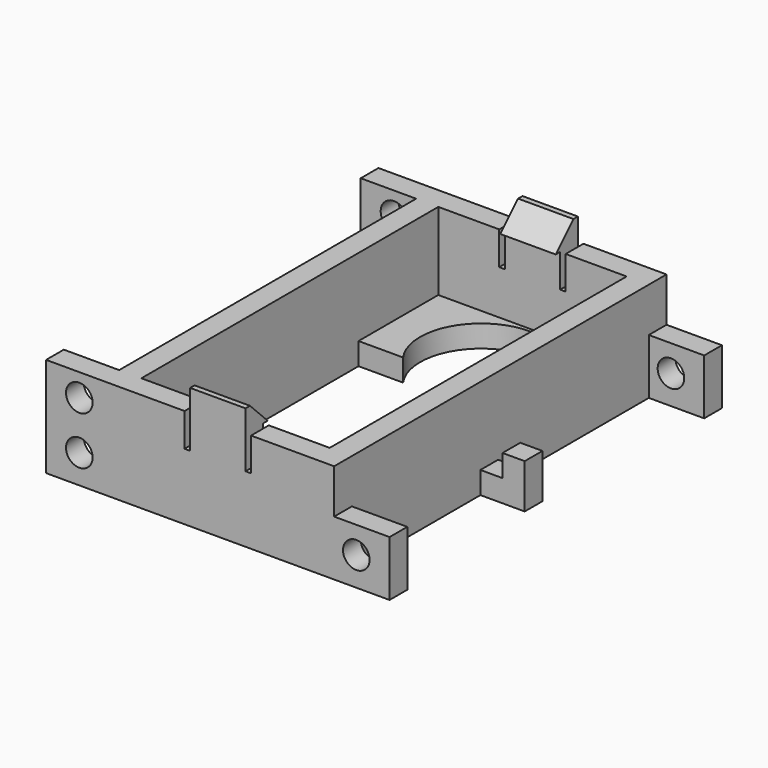
from build123d import *

# Parameters (mm, degrees)
F1_DEPTH  = 2
F2_DEPTH  = 9
F3_W      = 2
F3_H      = 5
F3_H_2    = 4
F4_DEPTH  = 5
F5_W      = 2
F5_H      = 5
F6_DEPTH  = 5
F7_R      = 1.2
F8_DEPTH  = 40
F11_DEPTH = 1
F12_W     = 5
F12_H     = 2
F12_H_2   = 0.5
F13_DEPTH = 2
F14_SIZE  = 1.99999
F12_W_2   = 0.5
F15_DEPTH = 3


# Not quite as in the source:
# - a fillet or chamfer is up to 0.001 mm smaller than in the source, because OpenCascade refuses the exact size


with BuildPart() as f1:
    # F0 (on Top) → F1 (new body)
    with BuildSketch(Plane.XY):
        Polygon((-5.1606558692, 9.7513413054), (-11.6606558692, 9.7513413054), (-11.6606558692, -27.7486586946), (-5.1606558692, -27.7486586946), (2.8393441308, -27.7486586946), (9.3393441308, -27.7486586946), (9.3393441308, 9.7513413054), (2.8393441308, 9.7513413054), align=None)
        Polygon((-9.6606558692, -1.2486586946), (-9.6606558692, 7.7513413054), (7.3393441308, 7.7513413054), (7.3393441308, -1.2486586946), (7.3393441308, -16.7486586946), (7.3393441308, -25.7486586946), (-9.6606558692, -25.7486586946), (-9.6606558692, -16.7486586946), align=None, mode=Mode.SUBTRACT)
        with BuildLine():
            Line((7.3393441308, 7.7513413054), (-9.6606558692, 7.7513413054))
            Line((-9.6606558692, 7.7513413054), (-9.6606558692, -1.2486586946))
            Line((-9.6606558692, -1.2486586946), (-5.6339097184, -1.2486586946))
            ThreePointArc((-5.6339097184, -1.2486586946), (-2.8409986659, 7.1883679509), (4.3393441308, 1.9513413054))
            ThreePointArc((4.3393441308, 1.9513413054), (4.0763707763, 0.2709985087), (3.3125979801, -1.2486586946))
            Line((3.3125979801, -1.2486586946), (7.3393441308, -1.2486586946))
            Line((7.3393441308, -1.2486586946), (7.3393441308, 7.7513413054))
        make_face()
        with BuildLine():
            Line((-5.6339097184, -16.7486586946), (-9.6606558692, -16.7486586946))
            Line((-9.6606558692, -16.7486586946), (-9.6606558692, -25.7486586946))
            Line((-9.6606558692, -25.7486586946), (7.3393441308, -25.7486586946))
            Line((7.3393441308, -25.7486586946), (7.3393441308, -16.7486586946))
            Line((7.3393441308, -16.7486586946), (3.3125979801, -16.7486586946))
            ThreePointArc((3.3125979801, -16.7486586946), (4.0763707763, -18.2683158979), (4.3393441308, -19.9486586946))
            ThreePointArc((4.3393441308, -19.9486586946), (-2.8409986659, -25.1856853401), (-5.6339097184, -16.7486586946))
        make_face()
    extrude(amount=F1_DEPTH)

    # F0 (on Top) → F2 (join)
    with BuildSketch(Plane.XY):
        Polygon((-5.1606558692, 9.7513413054), (-11.6606558692, 9.7513413054), (-11.6606558692, -27.7486586946), (-5.1606558692, -27.7486586946), (2.8393441308, -27.7486586946), (9.3393441308, -27.7486586946), (9.3393441308, 9.7513413054), (2.8393441308, 9.7513413054), align=None)
        Polygon((-9.6606558692, -1.2486586946), (-9.6606558692, 7.7513413054), (7.3393441308, 7.7513413054), (7.3393441308, -1.2486586946), (7.3393441308, -16.7486586946), (7.3393441308, -25.7486586946), (-9.6606558692, -25.7486586946), (-9.6606558692, -16.7486586946), align=None, mode=Mode.SUBTRACT)
    extrude(amount=F2_DEPTH)

    # F3 (on face) → F4 (join)
    with BuildSketch(Plane(origin=(-11.6606558692, 0, 0), x_dir=(0, -1, 0), z_dir=(-1, 0, 0))):
        with Locations((-8.7513413054, 2.5)):
            Rectangle(F3_W, F3_H)
        with Locations((-8.7513413054, 7)):
            Rectangle(F3_W, F3_H_2)
        with Locations((26.7486586946, 2.5)):
            Rectangle(F3_W, F3_H)
        with Locations((26.7486586946, 7)):
            Rectangle(F3_W, F3_H_2)
    extrude(amount=F4_DEPTH)

    # F5 (on face) → F6 (join)
    with BuildSketch(Plane.YZ.offset(9.3393441308)):
        with Locations((-26.7486586946, 2.5)):
            Rectangle(F5_W, F5_H)
        with Locations((8.7513413054, 2.5)):
            Rectangle(F5_W, F5_H)
    extrude(amount=F6_DEPTH)

    # F7 (on face) → F8 (cut)
    with BuildSketch(Plane.XZ.offset(27.7486586946)):
        with Locations((-13.6606558692, 2.6015837211)):
            Circle(F7_R)
        with Locations((11.3393441308, 2.6015837211)):
            Circle(F7_R)
        with Locations((-13.6606558692, 6.9661107846)):
            Circle(F7_R)
    extrude(amount=-F8_DEPTH, mode=Mode.SUBTRACT)

    # F10 (on offset) → F11 (join, symmetric)
    with BuildSketch(Plane(origin=(0, -10.2486586946, 0), x_dir=(-1, 0, 0), z_dir=(0, 1, 0))):
        Polygon((-13.3393441308, 4), (-13.3393441308, 0), (-9.3393441308, 0), (-9.3393441308, 2), (-11.3393441308, 2), (-11.3393441308, 4), align=None)
    extrude(amount=F11_DEPTH, both=True)

    # F12 (on face) → F13 (join)
    with BuildSketch(Plane.XY.offset(9)):
        with Locations((-1.1606558692, -26.7486586946)):
            Rectangle(F12_W, F12_H)
        with Locations((-1.1606558692, -25.4986586946)):
            Rectangle(F12_W, F12_H_2)
        with Locations((-1.1606558692, 8.7513413054)):
            Rectangle(F12_W, F12_H)
        with Locations((-1.1606558692, 7.5013413054)):
            Rectangle(F12_W, F12_H_2)
    extrude(amount=F13_DEPTH)

    # F14 (size 2 in the source; OpenCascade refuses exactly that, so slightly less here)
    f14_edges = [f1.edges().sort_by_distance(p)[0] for p in [
        (-1.160656, -25.248659, 11),
        (-1.160656, 7.251341, 11),
    ]]
    chamfer(f14_edges, length=F14_SIZE)

    # F12 (on face) → F15 (cut)
    with BuildSketch(Plane.XY.offset(9)):
        with Locations((-3.9106558692, -26.7486586946)):
            Rectangle(F12_W_2, F12_H)
        with Locations((1.5893441308, -26.7486586946)):
            Rectangle(F12_W_2, F12_H)
        with Locations((1.5893441308, 8.7513413054)):
            Rectangle(F12_W_2, F12_H)
        with Locations((-3.9106558692, 8.7513413054)):
            Rectangle(F12_W_2, F12_H)
    extrude(amount=-F15_DEPTH, mode=Mode.SUBTRACT)


solid = f1.part
